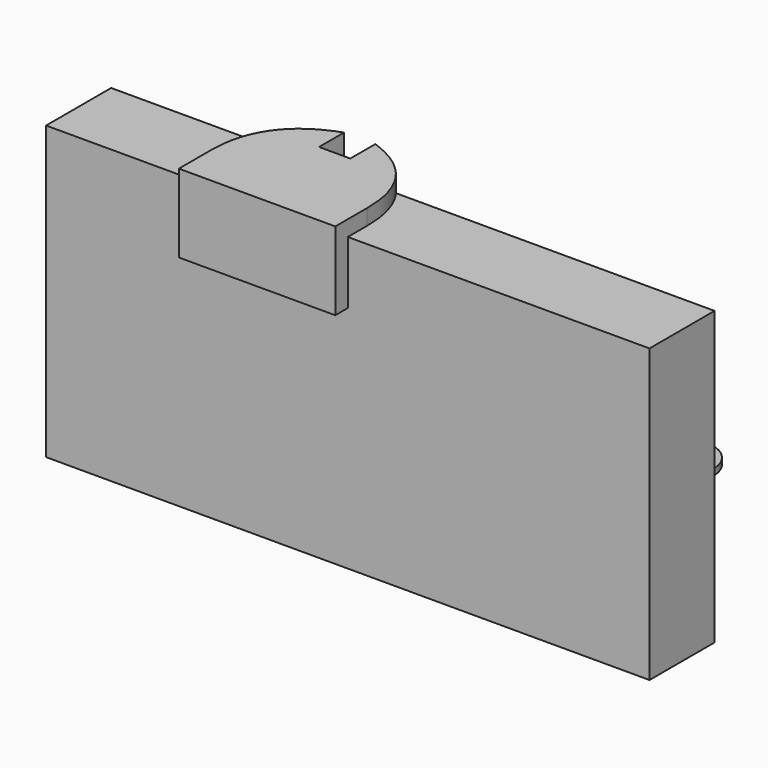
from build123d import *

# Parameters (mm, degrees)
F0_W        = 96.4427366853
F0_H        = 46.6602444649
F1_DEPTH    = 13
F2_W        = 10
F2_H        = 13
F2_H_2      = 2.5
F2_W_2      = 5
F3_DEPTH    = 2.5
F4_W        = 25
F4_H        = 2.5
F4_W_2      = 10
F4_H_2      = 5
F5_DEPTH    = 10
F6_T1_DEPTH = 83.2106781187
F6_T3_DEPTH = 83.2106781187
F8_DEPTH    = 1
F9_DEPTH    = 10
F10_R       = 5


# Not quite as in the source:
# - a fillet or chamfer that OpenCascade refuses, or shapes differently, is made with other operations: its cross-section is extruded or revolved along the edge and cut away or added


with BuildPart() as f1:
    # F0 (on Front) → F1 (new body)
    with BuildSketch(Plane.XZ):
        Rectangle(F0_W, F0_H)
    extrude(amount=F1_DEPTH)


with BuildPart() as f3:
    # F2 (on face) → F3 (new body)
    with BuildSketch(Plane.XY.offset(23.3301222324)):
        with Locations((-5, -6.5)):
            Rectangle(F2_W, F2_H)
        with Locations((-5, 1.25)):
            Rectangle(F2_W, F2_H_2)
        with Locations((-12.5, -6.5)):
            Rectangle(F2_W_2, F2_H)
        with Locations((-5, -14.25)):
            Rectangle(F2_W, F2_H_2)
        with Locations((-5, 3.75)):
            Rectangle(F2_W, F2_H_2)
        with Locations((-12.5, -14.25)):
            Rectangle(F2_W_2, F2_H_2)
        with Locations((-20, 1.25)):
            Rectangle(F2_W, F2_H_2)
        with Locations((-20, -6.5)):
            Rectangle(F2_W, F2_H)
        with Locations((-20, -14.25)):
            Rectangle(F2_W, F2_H_2)
        with Locations((-20, 3.75)):
            Rectangle(F2_W, F2_H_2)
    extrude(amount=F3_DEPTH)

    # F4 (on face) → F5 (join)
    with BuildSketch(Plane(origin=(0, 0, 23.3301222324), x_dir=(1, 0, 0), z_dir=(0, 0, -1))):
        with Locations((-12.5, 14.25)):
            Rectangle(F4_W, F4_H)
        with Locations((-20, -2.5)):
            Rectangle(F4_W_2, F4_H_2)
        with Locations((-5, -2.5)):
            Rectangle(F4_W_2, F4_H_2)
    extrude(amount=F5_DEPTH)

    # F6: fillet of radius 15 on 2 edges, made by hand

    # F6_s2 → F6_t1 (cut)
    with BuildSketch(Plane.XY.offset(-22.0252168269)):
        with BuildLine():
            add(Edge.make_bspline(
                [(-10, 5), (0, 1.4644660941), (0, -9.1421356237)],
                knots=[0, 0, 0, 1, 1, 1], degree=2, weights=[1, 1, 1]))
            Line((0, -9.1421356237), (0, 5))
            Line((0, 5), (-10, 5))
        make_face()
    extrude(amount=F6_T1_DEPTH, mode=Mode.SUBTRACT)

    # F6_s4 → F6_t3 (cut)
    with BuildSketch(Plane.XY.offset(-22.0252168269)):
        with BuildLine():
            add(Edge.make_bspline(
                [(-15, 5), (-25, 1.4644660941), (-25, -9.1421356237)],
                knots=[0, 0, 0, 1, 1, 1], degree=2, weights=[1, 1, 1]))
            Line((-25, -9.1421356237), (-25, 5))
            Line((-25, 5), (-15, 5))
        make_face()
    extrude(amount=F6_T3_DEPTH, mode=Mode.SUBTRACT)


with BuildPart() as f8:
    # F7 (on face) → F8 (new body)
    with BuildSketch(Plane(origin=(0, 0, -23.3301222324), x_dir=(1, 0, 0), z_dir=(0, 0, -1))):
        with BuildLine():
            Line((-15, -5), (-15, 0))
            Line((-15, 0), (-22.2784824925, 0))
            add(Edge.make_bspline(
                [(-22.2784824925, 0), (-20.6149497874, -2.2059261859), (-18.1887889565, -3.8725928525), (-15, -5)],
                knots=[0, 0, 0, 0, 1, 1, 1, 1], degree=3))
        make_face()
        Polygon((-10, 0), (-15, 0), (-15, -5), (-15, -40), (-10, -40), (-10, -5), align=None)
        with BuildLine():
            add(Edge.make_bspline(
                [(-22.2784824925, 0), (-20.6149497874, -2.2059261859), (-18.1887889565, -3.8725928525), (-15, -5)],
                knots=[0, 0, 0, 0, 1, 1, 1, 1], degree=3))
            Line((-22.2784824925, 0), (-45, 0))
            Line((-45, 0), (-45, -40))
            Line((-45, -40), (-15, -40))
            Line((-15, -40), (-15, -5))
        make_face()
        with BuildLine():
            Line((-2.7215175075, 0), (-10, 0))
            Line((-10, 0), (-10, -5))
            add(Edge.make_bspline(
                [(-10, -5), (-6.8112110435, -3.8725928525), (-4.3850502126, -2.2059261859), (-2.7215175075, 0)],
                knots=[0, 0, 0, 0, 1, 1, 1, 1], degree=3))
        make_face()
        with BuildLine():
            add(Edge.make_bspline(
                [(-10, -5), (-6.8112110435, -3.8725928525), (-4.3850502126, -2.2059261859), (-2.7215175075, 0)],
                knots=[0, 0, 0, 0, 1, 1, 1, 1], degree=3))
            Line((-10, -5), (-10, -40))
            Line((-10, -40), (20, -40))
            Line((20, -40), (20, 0))
            Line((20, 0), (-2.7215175075, 0))
        make_face()
    extrude(amount=-F8_DEPTH)

    # F7 (on face) → F9 (join)
    with BuildSketch(Plane(origin=(0, 0, -23.3301222324), x_dir=(1, 0, 0), z_dir=(0, 0, -1))):
        with BuildLine():
            Line((-2.7215175075, 0), (-10, 0))
            Line((-10, 0), (-10, -5))
            add(Edge.make_bspline(
                [(-10, -5), (-6.8112110435, -3.8725928525), (-4.3850502126, -2.2059261859), (-2.7215175075, 0)],
                knots=[0, 0, 0, 0, 1, 1, 1, 1], degree=3))
        make_face()
        with BuildLine():
            Line((-15, -5), (-15, 0))
            Line((-15, 0), (-22.2784824925, 0))
            add(Edge.make_bspline(
                [(-22.2784824925, 0), (-20.6149497874, -2.2059261859), (-18.1887889565, -3.8725928525), (-15, -5)],
                knots=[0, 0, 0, 0, 1, 1, 1, 1], degree=3))
        make_face()
    extrude(amount=-F9_DEPTH)

    # F10
    f10_edges = [f8.edges().sort_by_distance(p)[0] for p in [
        (20, 40, -22.830122),
        (-45, 40, -22.830122),
    ]]
    fillet(f10_edges, radius=F10_R)


solid = Compound([f1.part, f3.part, f8.part])
